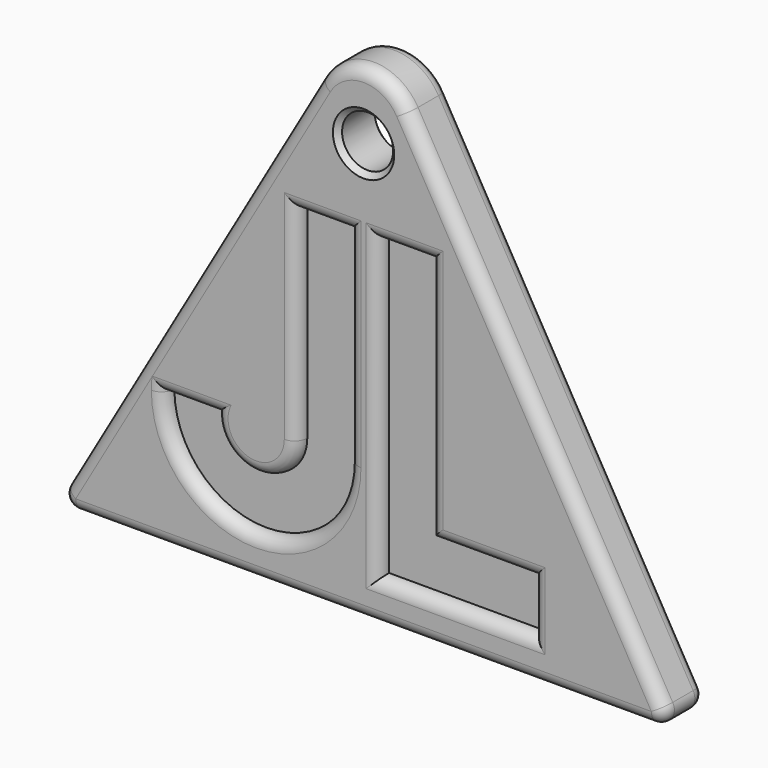
from build123d import *

# Parameters (mm, degrees)
F2_DEPTH      = 10
F3_START      = 7.5
F1_W          = 20
F1_H          = 10
F3_DEPTH      = 17.5
F4_W          = 20
F4_H          = 10
F5_DEPTH      = 2.5
F6_T1_DEPTH   = 5
F6_T3_DEPTH   = 123.1634295109
F6_T5_DEPTH   = 112.583302492
F6_T7_DEPTH   = 123.1634295109
F6_T9_DEPTH   = 54.25
F6_T11_DEPTH  = 26.25
F6_T13_DEPTH  = 10
F6_T15_DEPTH  = 30
F6_T17_DEPTH  = 58
F6_T19_DEPTH  = 10
F6_T21_DEPTH  = 40
F6_T23_DEPTH  = 10
F6_T25_DEPTH  = 30
F6_T27_DEPTH  = 26.25
F6_T32_DEPTH  = 2.5
F6_T38_DEPTH  = 2.5
F6_T44_DEPTH  = 2.5
F6_T50_DEPTH  = 2.5
F6_T56_DEPTH  = 16.25
F6_T61_DEPTH  = 22.5
F6_S62_R      = 8
F6_T63_DEPTH  = 13
F6_S64_R      = 18
F6_T65_DEPTH  = 13
F6_T67_ANGLE  = 180
F6_T71_DEPTH  = 16.25
F6_T74_ANGLE  = 180
F6_T78_DEPTH  = 16.25
F6_T81_ANGLE  = 180
F6_T85_DEPTH  = 22.5
F6_S86_R      = 8
F6_T87_DEPTH  = 13
F6_S88_R      = 18
F6_T89_DEPTH  = 13
F6_T91_ANGLE  = 180
F6_T95_DEPTH  = 16.25
F6_T101_DEPTH = 60.5
F6_T105_DEPTH = 16.25
F6_T112_DEPTH = 32.5
F6_T116_DEPTH = 16.25
F6_T123_DEPTH = 16.25
F6_T127_DEPTH = 36.25
F6_T134_DEPTH = 36.25
F6_T138_DEPTH = 64.25
F6_T145_DEPTH = 64.25
F6_T149_DEPTH = 16.25
F6_T157_DEPTH = 22.5
F6_S158_R     = 8
F6_T159_DEPTH = 13
F6_T162_ANGLE = 224.8343140314
F6_T169_DEPTH = 22.5
F6_S170_R     = 18
F6_T171_DEPTH = 13
F6_T174_ANGLE = 199.9263617918
F6_T181_DEPTH = 46.25
F6_T185_DEPTH = 16.25
F6_T192_DEPTH = 16.25
F6_T197_DEPTH = 46.25
F6_T204_DEPTH = 46.25
F6_T208_DEPTH = 16.25
F6_T216_DEPTH = 16.25
F6_T220_DEPTH = 46.25
F6_T227_ANGLE = 224.8343140314
F6_T231_DEPTH = 22.5
F6_S232_R     = 8
F6_T233_DEPTH = 13
F6_T239_DEPTH = 22.5
F6_S240_R     = 18
F6_T241_DEPTH = 13
F6_T244_ANGLE = 199.9263617918
F6_T251_DEPTH = 64.25
F6_T255_DEPTH = 36.25
F6_T262_DEPTH = 64.25
F6_T266_DEPTH = 16.25
F6_T274_DEPTH = 36.25
F6_T278_DEPTH = 16.25
F6_T285_DEPTH = 16.25
F6_T289_DEPTH = 32.5
F6_T296_DEPTH = 60.5
F6_T300_DEPTH = 16.25
F7_R          = 5
F8_DEPTH      = 25
F9_SIZE       = 1
F10_T1_DEPTH  = 9.9999999998
F10_T4_ANGLE  = 120
F10_T6_ANGLE  = 120


# Not quite as in the source:
# - a fillet or chamfer that OpenCascade refuses, or shapes differently, is made with other operations: its cross-section is extruded or revolved along the edge and cut away or added


with BuildPart() as f2:
    # F0 (on Front) → F2 (new body)
    with BuildSketch(Plane.XZ):
        Polygon((60.6217782649, -35), (0, 70), (-60.6217782649, -35), align=None)
    extrude(amount=F2_DEPTH)

    # F1 (on Front) → F3 (cut)
    with BuildSketch(Plane.XZ.offset(F3_START)):
        with BuildLine():
            ThreePointArc((-39, -9), (-21, -27), (-3, -9))
            Line((-3, -9), (-3, 31))
            Line((-3, 31), (-13, 31))
            Line((-13, 31), (-13, -9))
            ThreePointArc((-13, -9), (-21, -17), (-29, -9))
            Line((-29, -9), (-39, -9))
        make_face()
        Polygon((13, 31), (3, 31), (3, -27), (13, -27), (13, -17), align=None)
        with Locations((23, -22)):
            Rectangle(F1_W, F1_H)
    extrude(amount=F3_DEPTH, mode=Mode.SUBTRACT)

    # F4 (on face) → F5 (cut)
    with BuildSketch(Plane(origin=(0, 0, 0), x_dir=(-1, 0, 0), z_dir=(0, 1, 0))):
        with BuildLine():
            ThreePointArc((-39, -9), (-21, -27), (-3, -9))
            Line((-3, -9), (-3, 31))
            Line((-3, 31), (-13, 31))
            Line((-13, 31), (-13, -9))
            ThreePointArc((-13, -9), (-21, -17), (-29, -9))
            Line((-29, -9), (-39, -9))
        make_face()
        Polygon((13, 31), (3, 31), (3, -27), (13, -27), (13, -17), align=None)
        with Locations((23, -22)):
            Rectangle(F4_W, F4_H)
    extrude(amount=-F5_DEPTH, mode=Mode.SUBTRACT)

    # F6: fillet of radius 2.5 on 32 edges, made by hand

    # F6_s2 → F6_t1 (cut)
    with BuildSketch(Plane.XZ.offset(2.5)):
        with BuildLine():
            ThreePointArc((58.4567147554, -31.25), (58.4567147554, -33.75), (56.291651246, -35))
            Line((56.291651246, -35), (60.6217782649, -35))
            Line((60.6217782649, -35), (58.4567147554, -31.25))
        make_face()
        with BuildLine():
            ThreePointArc((-56.291651246, -35), (-58.4567147554, -33.75), (-58.4567147554, -31.25))
            Line((-58.4567147554, -31.25), (-60.6217782649, -35))
            Line((-60.6217782649, -35), (-56.291651246, -35))
        make_face()
    extrude(amount=F6_T1_DEPTH, mode=Mode.SUBTRACT)

    # F6_s4 → F6_t3 (cut)
    with BuildSketch(Plane(origin=(28.145825623, 0, -48.75), x_dir=(0, 1, 0), z_dir=(-0.5, 0, 0.8660254038))):
        with BuildLine():
            ThreePointArc((-2.5, -35), (-0.732233047, -34.267766953), (0, -32.5))
            Line((0, -32.5), (0, -35))
            Line((0, -35), (-2.5, -35))
        make_face()
        with BuildLine():
            ThreePointArc((-7.5, -35), (-9.267766953, -34.267766953), (-10, -32.5))
            Line((-10, -32.5), (-10, -35))
            Line((-10, -35), (-7.5, -35))
        make_face()
    extrude(amount=F6_T3_DEPTH, mode=Mode.SUBTRACT)

    # F6_s6 → F6_t5 (cut)
    with BuildSketch(Plane.YZ.offset(-56.291651246)):
        with BuildLine():
            ThreePointArc((-2.5, -35), (-0.732233047, -34.267766953), (0, -32.5))
            Line((0, -32.5), (0, -35))
            Line((0, -35), (-2.5, -35))
        make_face()
        with BuildLine():
            ThreePointArc((-7.5, -35), (-9.267766953, -34.267766953), (-10, -32.5))
            Line((-10, -32.5), (-10, -35))
            Line((-10, -35), (-7.5, -35))
        make_face()
    extrude(amount=F6_T5_DEPTH, mode=Mode.SUBTRACT)

    # F6_s8 → F6_t7 (cut)
    with BuildSketch(Plane(origin=(33.4358891325, 0, 57.9126587737), x_dir=(0, 1, 0), z_dir=(-0.5, 0, -0.8660254038))):
        with BuildLine():
            ThreePointArc((-2.5, -35), (-0.732233047, -34.267766953), (0, -32.5))
            Line((0, -32.5), (0, -35))
            Line((0, -35), (-2.5, -35))
        make_face()
        with BuildLine():
            ThreePointArc((-7.5, -35), (-9.267766953, -34.267766953), (-10, -32.5))
            Line((-10, -32.5), (-10, -35))
            Line((-10, -35), (-7.5, -35))
        make_face()
    extrude(amount=F6_T7_DEPTH, mode=Mode.SUBTRACT)

    # F6_s10 → F6_t9 (cut)
    with BuildSketch(Plane.XY.offset(-23.25)):
        with BuildLine():
            ThreePointArc((-15.5, 0), (-13.732233047, -0.732233047), (-13, -2.5))
            Line((-13, -2.5), (-13, 0))
            Line((-13, 0), (-15.5, 0))
        make_face()
        with BuildLine():
            ThreePointArc((15.5, -10), (13.732233047, -9.267766953), (13, -7.5))
            Line((13, -7.5), (13, -10))
            Line((13, -10), (15.5, -10))
        make_face()
    extrude(amount=F6_T9_DEPTH, mode=Mode.SUBTRACT)

    # F6_s12 → F6_t11 (cut)
    with BuildSketch(Plane.YZ.offset(-33)):
        with BuildLine():
            ThreePointArc((0, -14.5), (-0.732233047, -16.267766953), (-2.5, -17))
            Line((-2.5, -17), (0, -17))
            Line((0, -17), (0, -14.5))
        make_face()
    extrude(amount=F6_T11_DEPTH, mode=Mode.SUBTRACT)

    # F6_s14 → F6_t13 (cut)
    with BuildSketch(Plane.XY.offset(-27)):
        with BuildLine():
            ThreePointArc((-35.5, 0), (-33.732233047, -0.732233047), (-33, -2.5))
            Line((-33, -2.5), (-33, 0))
            Line((-33, 0), (-35.5, 0))
        make_face()
        with BuildLine():
            ThreePointArc((35.5, -10), (33.732233047, -9.267766953), (33, -7.5))
            Line((33, -7.5), (33, -10))
            Line((33, -10), (35.5, -10))
        make_face()
    extrude(amount=F6_T13_DEPTH, mode=Mode.SUBTRACT)

    # F6_s16 → F6_t15 (cut)
    with BuildSketch(Plane.YZ.offset(-33)):
        with BuildLine():
            ThreePointArc((0, -29.5), (-0.732233047, -27.732233047), (-2.5, -27))
            Line((-2.5, -27), (0, -27))
            Line((0, -27), (0, -29.5))
        make_face()
    extrude(amount=F6_T15_DEPTH, mode=Mode.SUBTRACT)

    # F6_s18 → F6_t17 (cut)
    with BuildSketch(Plane.XY.offset(-27)):
        with BuildLine():
            ThreePointArc((-0.5, 0), (-2.267766953, -0.732233047), (-3, -2.5))
            Line((-3, -2.5), (-3, 0))
            Line((-3, 0), (-0.5, 0))
        make_face()
        with BuildLine():
            ThreePointArc((0.5, -10), (2.267766953, -9.267766953), (3, -7.5))
            Line((3, -7.5), (3, -10))
            Line((3, -10), (0.5, -10))
        make_face()
    extrude(amount=F6_T17_DEPTH, mode=Mode.SUBTRACT)

    # F6_s20 → F6_t19 (cut)
    with BuildSketch(Plane.YZ.offset(-13)):
        with BuildLine():
            ThreePointArc((0, 33.5), (-0.732233047, 31.732233047), (-2.5, 31))
            Line((-2.5, 31), (0, 31))
            Line((0, 31), (0, 33.5))
        make_face()
        with BuildLine():
            ThreePointArc((-10, 33.5), (-9.267766953, 31.732233047), (-7.5, 31))
            Line((-7.5, 31), (-10, 31))
            Line((-10, 31), (-10, 33.5))
        make_face()
    extrude(amount=F6_T19_DEPTH, mode=Mode.SUBTRACT)

    # F6_s22 → F6_t21 (cut)
    with BuildSketch(Plane.XY.offset(-9)):
        with BuildLine():
            ThreePointArc((15.5, 0), (13.732233047, -0.732233047), (13, -2.5))
            Line((13, -2.5), (13, 0))
            Line((13, 0), (15.5, 0))
        make_face()
        with BuildLine():
            ThreePointArc((0.5, 0), (2.267766953, -0.732233047), (3, -2.5))
            Line((3, -2.5), (3, 0))
            Line((3, 0), (0.5, 0))
        make_face()
        with BuildLine():
            ThreePointArc((-0.5, -10), (-2.267766953, -9.267766953), (-3, -7.5))
            Line((-3, -7.5), (-3, -10))
            Line((-3, -10), (-0.5, -10))
        make_face()
        with BuildLine():
            ThreePointArc((-15.5, -10), (-13.732233047, -9.267766953), (-13, -7.5))
            Line((-13, -7.5), (-13, -10))
            Line((-13, -10), (-15.5, -10))
        make_face()
    extrude(amount=F6_T21_DEPTH, mode=Mode.SUBTRACT)

    # F6_s24 → F6_t23 (cut)
    with BuildSketch(Plane.YZ.offset(3)):
        with BuildLine():
            ThreePointArc((0, 33.5), (-0.732233047, 31.732233047), (-2.5, 31))
            Line((-2.5, 31), (0, 31))
            Line((0, 31), (0, 33.5))
        make_face()
        with BuildLine():
            ThreePointArc((-10, 33.5), (-9.267766953, 31.732233047), (-7.5, 31))
            Line((-7.5, 31), (-10, 31))
            Line((-10, 31), (-10, 33.5))
        make_face()
    extrude(amount=F6_T23_DEPTH, mode=Mode.SUBTRACT)

    # F6_s26 → F6_t25 (cut)
    with BuildSketch(Plane.YZ.offset(3)):
        with BuildLine():
            ThreePointArc((-10, -29.5), (-9.267766953, -27.732233047), (-7.5, -27))
            Line((-7.5, -27), (-10, -27))
            Line((-10, -27), (-10, -29.5))
        make_face()
    extrude(amount=F6_T25_DEPTH, mode=Mode.SUBTRACT)

    # F6_s28 → F6_t27 (cut)
    with BuildSketch(Plane.YZ.offset(6.75)):
        with BuildLine():
            ThreePointArc((-10, -14.5), (-9.267766953, -16.267766953), (-7.5, -17))
            Line((-7.5, -17), (-10, -17))
            Line((-10, -17), (-10, -14.5))
        make_face()
    extrude(amount=F6_T27_DEPTH, mode=Mode.SUBTRACT)


with BuildPart() as f6_tool30:
    # F6_s31 → F6_t32 (new body)
    with BuildSketch(Plane.XZ.offset(2.5)):
        Polygon((56.291651246, -32.5), (58.4567147554, -31.25), (60.6217782649, -35), (56.291651246, -35), align=None)
    extrude(amount=-F6_T32_DEPTH)

    # F6_s33 → F6_t34 (revolve, cut)
    with BuildSketch(Plane(origin=(56.291651246, -2.5, -32.5), x_dir=(-0.8660254038, 0, 0.5), z_dir=(-0.5, 0, -0.8660254038))):
        with BuildLine():
            ThreePointArc((0, -2.5), (2.5, 0), (0, 2.5))
            Line((0, 2.5), (0, -2.5))
        make_face()
    revolve(axis=Axis((56.291651246, -2.5, -32.5), (0, 1, 0)), mode=Mode.SUBTRACT)


with BuildPart() as f2_1:
    add(f2.part)

    # F6_t29: cut F6_tool30
    add(f6_tool30.part, mode=Mode.SUBTRACT)


with BuildPart() as f6_tool36:
    # F6_s37 → F6_t38 (new body)
    with BuildSketch(Plane.XZ.offset(7.5)):
        Polygon((56.291651246, -32.5), (58.4567147554, -31.25), (60.6217782649, -35), (56.291651246, -35), align=None)
    extrude(amount=F6_T38_DEPTH)

    # F6_s39 → F6_t40 (revolve, cut)
    with BuildSketch(Plane(origin=(56.291651246, -7.5, -32.5), x_dir=(-0.8660254038, 0, 0.5), z_dir=(0.5, 0, 0.8660254038))):
        with BuildLine():
            ThreePointArc((0, -2.5), (2.5, 0), (0, 2.5))
            Line((0, 2.5), (0, -2.5))
        make_face()
    revolve(axis=Axis((56.291651246, -7.5, -32.5), (0, -1, 0)), mode=Mode.SUBTRACT)


with BuildPart() as f2_2:
    add(f2_1.part)

    # F6_t35: cut F6_tool36
    add(f6_tool36.part, mode=Mode.SUBTRACT)


with BuildPart() as f6_tool42:
    # F6_s43 → F6_t44 (new body)
    with BuildSketch(Plane.XZ.offset(2.5)):
        Polygon((-56.291651246, -32.5), (-56.291651246, -35), (-60.6217782649, -35), (-58.4567147554, -31.25), align=None)
    extrude(amount=-F6_T44_DEPTH)

    # F6_s45 → F6_t46 (revolve, cut)
    with BuildSketch(Plane(origin=(-56.291651246, -2.5, -32.5), x_dir=(0.8660254038, 0, 0.5), z_dir=(-0.5, 0, 0.8660254038))):
        with BuildLine():
            ThreePointArc((0, -2.5), (2.5, 0), (0, 2.5))
            Line((0, 2.5), (0, -2.5))
        make_face()
    revolve(axis=Axis((-56.291651246, -2.5, -32.5), (0, 1, 0)), mode=Mode.SUBTRACT)


with BuildPart() as f2_3:
    add(f2_2.part)

    # F6_t41: cut F6_tool42
    add(f6_tool42.part, mode=Mode.SUBTRACT)


with BuildPart() as f6_tool48:
    # F6_s49 → F6_t50 (new body)
    with BuildSketch(Plane.XZ.offset(7.5)):
        Polygon((-56.291651246, -32.5), (-56.291651246, -35), (-60.6217782649, -35), (-58.4567147554, -31.25), align=None)
    extrude(amount=F6_T50_DEPTH)

    # F6_s51 → F6_t52 (revolve, cut)
    with BuildSketch(Plane(origin=(-56.291651246, -7.5, -32.5), x_dir=(0.8660254038, 0, 0.5), z_dir=(0.5, 0, -0.8660254038))):
        with BuildLine():
            ThreePointArc((0, -2.5), (2.5, 0), (0, 2.5))
            Line((0, 2.5), (0, -2.5))
        make_face()
    revolve(axis=Axis((-56.291651246, -7.5, -32.5), (0, -1, 0)), mode=Mode.SUBTRACT)


with BuildPart() as f2_4:
    add(f2_3.part)

    # F6_t47: cut F6_tool48
    add(f6_tool48.part, mode=Mode.SUBTRACT)


with BuildPart() as f6_tool54:
    # F6_s55 → F6_t56 (new body)
    with BuildSketch(Plane.YZ.offset(-13)):
        with BuildLine():
            ThreePointArc((0, 33.5), (-0.732233047, 31.732233047), (-2.5, 31))
            Line((-2.5, 31), (0, 31))
            Line((0, 31), (0, 33.5))
        make_face()
    extrude(amount=F6_T56_DEPTH)

    split(bisect_by=Plane.YZ.offset(3), keep=Keep.TOP)


with BuildPart() as f2_5:
    add(f2_4.part)

    # F6_t53: cut F6_tool54
    add(f6_tool54.part, mode=Mode.SUBTRACT)


with BuildPart() as f6_tool59:
    # F6_s60 → F6_t61 (new body)
    with BuildSketch(Plane.YZ.offset(22.75)):
        with BuildLine():
            ThreePointArc((0, -6.5), (-0.732233047, -8.267766953), (-2.5, -9))
            Line((-2.5, -9), (0, -9))
            Line((0, -9), (0, -6.5))
        make_face()
    extrude(amount=F6_T61_DEPTH)

    # F6_s62 → F6_t63 (cut, symmetric)
    with BuildSketch(Plane.XZ.offset(1.2)):
        with Locations((21, -9)):
            Circle(F6_S62_R)
    extrude(amount=F6_T63_DEPTH, both=True, mode=Mode.SUBTRACT)

    # F6_s64 → F6_t65 (intersect, symmetric)
    with BuildSketch(Plane.XZ.offset(1.2)):
        with Locations((21, -9)):
            Circle(F6_S64_R)
    extrude(amount=F6_T65_DEPTH, both=True, mode=Mode.INTERSECT)


with BuildPart() as f2_6:
    add(f2_5.part)

    # F6_t58: cut F6_tool59
    add(f6_tool59.part, mode=Mode.SUBTRACT)

    # F6_s66 → F6_t67 (revolve, cut)
    with BuildSketch(Plane.XY.offset(-9)):
        with BuildLine():
            ThreePointArc((15.5, 0), (13.732233047, -0.732233047), (13, -2.5))
            Line((13, -2.5), (13, 0))
            Line((13, 0), (15.5, 0))
        make_face()
    revolve(axis=Axis((21, 0, -9), (0, -1, 0)), revolution_arc=F6_T67_ANGLE, mode=Mode.SUBTRACT)


with BuildPart() as f6_tool69:
    # F6_s70 → F6_t71 (new body)
    with BuildSketch(Plane.YZ.offset(-3.25)):
        with BuildLine():
            ThreePointArc((0, 33.5), (-0.732233047, 31.732233047), (-2.5, 31))
            Line((-2.5, 31), (0, 31))
            Line((0, 31), (0, 33.5))
        make_face()
    extrude(amount=F6_T71_DEPTH)

    split(bisect_by=Plane.YZ.offset(-3), keep=Keep.BOTTOM)


with BuildPart() as f2_7:
    add(f2_6.part)

    # F6_t68: cut F6_tool69
    add(f6_tool69.part, mode=Mode.SUBTRACT)

    # F6_s73 → F6_t74 (revolve, cut)
    with BuildSketch(Plane.XY.offset(-9)):
        with BuildLine():
            ThreePointArc((41.5, 0), (39.732233047, -0.732233047), (39, -2.5))
            Line((39, -2.5), (39, 0))
            Line((39, 0), (41.5, 0))
        make_face()
    revolve(axis=Axis((21, 0, -9), (0, 1, 0)), revolution_arc=F6_T74_ANGLE, mode=Mode.SUBTRACT)


with BuildPart() as f6_tool76:
    # F6_s77 → F6_t78 (new body)
    with BuildSketch(Plane.YZ.offset(-13)):
        with BuildLine():
            ThreePointArc((-10, 33.5), (-9.267766953, 31.732233047), (-7.5, 31))
            Line((-7.5, 31), (-10, 31))
            Line((-10, 31), (-10, 33.5))
        make_face()
    extrude(amount=F6_T78_DEPTH)

    split(bisect_by=Plane.YZ.offset(3), keep=Keep.TOP)


with BuildPart() as f2_8:
    add(f2_7.part)

    # F6_t75: cut F6_tool76
    add(f6_tool76.part, mode=Mode.SUBTRACT)

    # F6_s80 → F6_t81 (revolve, cut)
    with BuildSketch(Plane.XY.offset(-9)):
        with BuildLine():
            ThreePointArc((-15.5, -10), (-13.732233047, -9.267766953), (-13, -7.5))
            Line((-13, -7.5), (-13, -10))
            Line((-13, -10), (-15.5, -10))
        make_face()
    revolve(axis=Axis((-21, -10, -9), (0, 1, 0)), revolution_arc=F6_T81_ANGLE, mode=Mode.SUBTRACT)


with BuildPart() as f6_tool83:
    # F6_s84 → F6_t85 (new body)
    with BuildSketch(Plane.YZ.offset(-45.25)):
        with BuildLine():
            ThreePointArc((-10, -6.5), (-9.267766953, -8.267766953), (-7.5, -9))
            Line((-7.5, -9), (-10, -9))
            Line((-10, -9), (-10, -6.5))
        make_face()
    extrude(amount=F6_T85_DEPTH)

    # F6_s86 → F6_t87 (cut, symmetric)
    with BuildSketch(Plane.XZ.offset(8.8)):
        with Locations((-21, -9)):
            Circle(F6_S86_R)
    extrude(amount=F6_T87_DEPTH, both=True, mode=Mode.SUBTRACT)

    # F6_s88 → F6_t89 (intersect, symmetric)
    with BuildSketch(Plane.XZ.offset(8.8)):
        with Locations((-21, -9)):
            Circle(F6_S88_R)
    extrude(amount=F6_T89_DEPTH, both=True, mode=Mode.INTERSECT)


with BuildPart() as f2_9:
    add(f2_8.part)

    # F6_t82: cut F6_tool83
    add(f6_tool83.part, mode=Mode.SUBTRACT)

    # F6_s90 → F6_t91 (revolve, cut)
    with BuildSketch(Plane.XY.offset(-9)):
        with BuildLine():
            ThreePointArc((-0.5, -10), (-2.267766953, -9.267766953), (-3, -7.5))
            Line((-3, -7.5), (-3, -10))
            Line((-3, -10), (-0.5, -10))
        make_face()
    revolve(axis=Axis((-21, -10, -9), (0, 1, 0)), revolution_arc=F6_T91_ANGLE, mode=Mode.SUBTRACT)


with BuildPart() as f6_tool93:
    # F6_s94 → F6_t95 (new body)
    with BuildSketch(Plane.YZ.offset(-3.25)):
        with BuildLine():
            ThreePointArc((-10, 33.5), (-9.267766953, 31.732233047), (-7.5, 31))
            Line((-7.5, 31), (-10, 31))
            Line((-10, 31), (-10, 33.5))
        make_face()
    extrude(amount=F6_T95_DEPTH)

    split(bisect_by=Plane.YZ.offset(-3), keep=Keep.BOTTOM)


with BuildPart() as f2_10:
    add(f2_9.part)

    # F6_t92: cut F6_tool93
    add(f6_tool93.part, mode=Mode.SUBTRACT)


with BuildPart() as f6_tool99:
    # F6_s100 → F6_t101 (new body)
    with BuildSketch(Plane.XY.offset(-23.25)):
        with BuildLine():
            ThreePointArc((-15.5, 0), (-13.732233047, -0.732233047), (-13, -2.5))
            Line((-13, -2.5), (-13, 0))
            Line((-13, 0), (-15.5, 0))
        make_face()
    extrude(amount=F6_T101_DEPTH)

    split(bisect_by=Plane.XY.offset(31), keep=Keep.TOP)


with BuildPart() as f6_tool103:
    # F6_s104 → F6_t105 (new body)
    with BuildSketch(Plane.YZ.offset(-19.25)):
        with BuildLine():
            ThreePointArc((0, 33.5), (-0.732233047, 31.732233047), (-2.5, 31))
            Line((-2.5, 31), (0, 31))
            Line((0, 31), (0, 33.5))
        make_face()
    extrude(amount=F6_T105_DEPTH)

    split(bisect_by=Plane.YZ.offset(-13), keep=Keep.BOTTOM)


with BuildPart() as f6_tool99_1:
    add(f6_tool99.part)

    # F6_t107: intersect F6_tool103
    add(f6_tool103.part, mode=Mode.INTERSECT)


with BuildPart() as f2_11:
    add(f2_10.part)

    # F6_t97: cut F6_tool99
    add(f6_tool99_1.part, mode=Mode.SUBTRACT)


with BuildPart() as f6_tool110:
    # F6_s111 → F6_t112 (new body)
    with BuildSketch(Plane.YZ.offset(-39.25)):
        with BuildLine():
            ThreePointArc((0, -14.5), (-0.732233047, -16.267766953), (-2.5, -17))
            Line((-2.5, -17), (0, -17))
            Line((0, -17), (0, -14.5))
        make_face()
    extrude(amount=F6_T112_DEPTH)

    split(bisect_by=Plane.YZ.offset(-33), keep=Keep.BOTTOM)


with BuildPart() as f6_tool114:
    # F6_s115 → F6_t116 (new body)
    with BuildSketch(Plane.XY.offset(-27)):
        with BuildLine():
            ThreePointArc((-35.5, 0), (-33.732233047, -0.732233047), (-33, -2.5))
            Line((-33, -2.5), (-33, 0))
            Line((-33, 0), (-35.5, 0))
        make_face()
    extrude(amount=F6_T116_DEPTH)

    split(bisect_by=Plane.XY.offset(-17), keep=Keep.TOP)


with BuildPart() as f6_tool110_1:
    add(f6_tool110.part)

    # F6_t118: intersect F6_tool114
    add(f6_tool114.part, mode=Mode.INTERSECT)


with BuildPart() as f2_12:
    add(f2_11.part)

    # F6_t108: cut F6_tool110
    add(f6_tool110_1.part, mode=Mode.SUBTRACT)


with BuildPart() as f6_tool121:
    # F6_s122 → F6_t123 (new body)
    with BuildSketch(Plane.XY.offset(-33.25)):
        with BuildLine():
            ThreePointArc((-35.5, 0), (-33.732233047, -0.732233047), (-33, -2.5))
            Line((-33, -2.5), (-33, 0))
            Line((-33, 0), (-35.5, 0))
        make_face()
    extrude(amount=F6_T123_DEPTH)

    split(bisect_by=Plane.XY.offset(-27), keep=Keep.BOTTOM)


with BuildPart() as f6_tool125:
    # F6_s126 → F6_t127 (new body)
    with BuildSketch(Plane.YZ.offset(-3)):
        with BuildLine():
            ThreePointArc((0, -29.5), (-0.732233047, -27.732233047), (-2.5, -27))
            Line((-2.5, -27), (0, -27))
            Line((0, -27), (0, -29.5))
        make_face()
    extrude(amount=-F6_T127_DEPTH)

    split(bisect_by=Plane.YZ.offset(-33), keep=Keep.BOTTOM)


with BuildPart() as f6_tool121_1:
    add(f6_tool121.part)

    # F6_t129: intersect F6_tool125
    add(f6_tool125.part, mode=Mode.INTERSECT)


with BuildPart() as f2_13:
    add(f2_12.part)

    # F6_t119: cut F6_tool121
    add(f6_tool121_1.part, mode=Mode.SUBTRACT)


with BuildPart() as f6_tool132:
    # F6_s133 → F6_t134 (new body)
    with BuildSketch(Plane.YZ.offset(3.25)):
        with BuildLine():
            ThreePointArc((0, -29.5), (-0.732233047, -27.732233047), (-2.5, -27))
            Line((-2.5, -27), (0, -27))
            Line((0, -27), (0, -29.5))
        make_face()
    extrude(amount=-F6_T134_DEPTH)

    split(bisect_by=Plane.YZ.offset(-3), keep=Keep.TOP)


with BuildPart() as f6_tool136:
    # F6_s137 → F6_t138 (new body)
    with BuildSketch(Plane.XY.offset(31)):
        with BuildLine():
            ThreePointArc((-0.5, 0), (-2.267766953, -0.732233047), (-3, -2.5))
            Line((-3, -2.5), (-3, 0))
            Line((-3, 0), (-0.5, 0))
        make_face()
    extrude(amount=-F6_T138_DEPTH)

    split(bisect_by=Plane.XY.offset(-27), keep=Keep.BOTTOM)


with BuildPart() as f6_tool132_1:
    add(f6_tool132.part)

    # F6_t140: intersect F6_tool136
    add(f6_tool136.part, mode=Mode.INTERSECT)


with BuildPart() as f2_14:
    add(f2_13.part)

    # F6_t130: cut F6_tool132
    add(f6_tool132_1.part, mode=Mode.SUBTRACT)


with BuildPart() as f6_tool143:
    # F6_s144 → F6_t145 (new body)
    with BuildSketch(Plane.XY.offset(37.25)):
        with BuildLine():
            ThreePointArc((-0.5, 0), (-2.267766953, -0.732233047), (-3, -2.5))
            Line((-3, -2.5), (-3, 0))
            Line((-3, 0), (-0.5, 0))
        make_face()
    extrude(amount=-F6_T145_DEPTH)

    split(bisect_by=Plane.XY.offset(31), keep=Keep.TOP)


with BuildPart() as f6_tool147:
    # F6_s148 → F6_t149 (new body)
    with BuildSketch(Plane.YZ.offset(-13)):
        with BuildLine():
            ThreePointArc((0, 33.5), (-0.732233047, 31.732233047), (-2.5, 31))
            Line((-2.5, 31), (0, 31))
            Line((0, 31), (0, 33.5))
        make_face()
    extrude(amount=F6_T149_DEPTH)

    split(bisect_by=Plane.YZ.offset(-3), keep=Keep.TOP)

    split(bisect_by=Plane.YZ.offset(3), keep=Keep.BOTTOM)


with BuildPart() as f6_tool143_1:
    add(f6_tool143.part)

    # F6_t152: intersect F6_tool147
    add(f6_tool147.part, mode=Mode.INTERSECT)


with BuildPart() as f2_15:
    add(f2_14.part)

    # F6_t141: cut F6_tool143
    add(f6_tool143_1.part, mode=Mode.SUBTRACT)


with BuildPart() as f6_tool155:
    # F6_s156 → F6_t157 (new body)
    with BuildSketch(Plane.YZ.offset(22.75)):
        with BuildLine():
            ThreePointArc((0, -6.5), (-0.732233047, -8.267766953), (-2.5, -9))
            Line((-2.5, -9), (0, -9))
            Line((0, -9), (0, -6.5))
        make_face()
    extrude(amount=F6_T157_DEPTH)

    # F6_s158 → F6_t159 (intersect, symmetric)
    with BuildSketch(Plane.XZ.offset(1.2)):
        with Locations((21, -9)):
            Circle(F6_S158_R)
    extrude(amount=F6_T159_DEPTH, both=True, mode=Mode.INTERSECT)


with BuildPart() as f6_tool160:
    # F6_s161 → F6_t162 (revolve)
    with BuildSketch(Plane.XY.offset(-9)):
        with BuildLine():
            ThreePointArc((15.5, 0), (13.732233047, -0.732233047), (13, -2.5))
            Line((13, -2.5), (13, 0))
            Line((13, 0), (15.5, 0))
        make_face()
    revolve(axis=Axis((21, 0, -9), (0, -1, 0)), revolution_arc=F6_T162_ANGLE)

    split(bisect_by=Plane.XY.offset(-9), keep=Keep.TOP)


with BuildPart() as f6_tool155_1:
    add(f6_tool155.part)

    # F6_t164: intersect F6_tool160
    add(f6_tool160.part, mode=Mode.INTERSECT)


with BuildPart() as f2_16:
    add(f2_15.part)

    # F6_t153: cut F6_tool155
    add(f6_tool155_1.part, mode=Mode.SUBTRACT)


with BuildPart() as f6_tool167:
    # F6_s168 → F6_t169 (new body)
    with BuildSketch(Plane.YZ.offset(22.75)):
        with BuildLine():
            ThreePointArc((0, -6.5), (-0.732233047, -8.267766953), (-2.5, -9))
            Line((-2.5, -9), (0, -9))
            Line((0, -9), (0, -6.5))
        make_face()
    extrude(amount=F6_T169_DEPTH)

    # F6_s170 → F6_t171 (cut, symmetric)
    with BuildSketch(Plane.XZ.offset(1.2)):
        with Locations((21, -9)):
            Circle(F6_S170_R)
    extrude(amount=F6_T171_DEPTH, both=True, mode=Mode.SUBTRACT)


with BuildPart() as f6_tool172:
    # F6_s173 → F6_t174 (revolve)
    with BuildSketch(Plane(origin=(5.322885035, 0, -14.6831959933), x_dir=(0, 1, 0), z_dir=(-0.3408121408, 0, 0.9401314188))):
        with BuildLine():
            ThreePointArc((0, -37.1754505284), (-0.732233047, -35.4076835755), (-2.5, -34.6754505284))
            Line((-2.5, -34.6754505284), (0, -34.6754505284))
            Line((0, -34.6754505284), (0, -37.1754505284))
        make_face()
    revolve(axis=Axis((21, 0, -9), (0, 1, 0)), revolution_arc=F6_T174_ANGLE)

    split(bisect_by=Plane.XY.offset(-9), keep=Keep.TOP)


with BuildPart() as f6_tool167_1:
    add(f6_tool167.part)

    # F6_t176: intersect F6_tool172
    add(f6_tool172.part, mode=Mode.INTERSECT)


with BuildPart() as f2_17:
    add(f2_16.part)

    # F6_t165: cut F6_tool167
    add(f6_tool167_1.part, mode=Mode.SUBTRACT)


with BuildPart() as f6_tool179:
    # F6_s180 → F6_t181 (new body)
    with BuildSketch(Plane.XY.offset(37.25)):
        with BuildLine():
            ThreePointArc((15.5, 0), (13.732233047, -0.732233047), (13, -2.5))
            Line((13, -2.5), (13, 0))
            Line((13, 0), (15.5, 0))
        make_face()
    extrude(amount=-F6_T181_DEPTH)

    split(bisect_by=Plane.XY.offset(31), keep=Keep.TOP)


with BuildPart() as f6_tool183:
    # F6_s184 → F6_t185 (new body)
    with BuildSketch(Plane.YZ.offset(3)):
        with BuildLine():
            ThreePointArc((0, 33.5), (-0.732233047, 31.732233047), (-2.5, 31))
            Line((-2.5, 31), (0, 31))
            Line((0, 31), (0, 33.5))
        make_face()
    extrude(amount=F6_T185_DEPTH)

    split(bisect_by=Plane.YZ.offset(13), keep=Keep.TOP)


with BuildPart() as f6_tool179_1:
    add(f6_tool179.part)

    # F6_t187: intersect F6_tool183
    add(f6_tool183.part, mode=Mode.INTERSECT)


with BuildPart() as f2_18:
    add(f2_17.part)

    # F6_t177: cut F6_tool179
    add(f6_tool179_1.part, mode=Mode.SUBTRACT)


with BuildPart() as f6_tool190:
    # F6_s191 → F6_t192 (new body)
    with BuildSketch(Plane.YZ.offset(-3.25)):
        with BuildLine():
            ThreePointArc((0, 33.5), (-0.732233047, 31.732233047), (-2.5, 31))
            Line((-2.5, 31), (0, 31))
            Line((0, 31), (0, 33.5))
        make_face()
    extrude(amount=F6_T192_DEPTH)

    split(bisect_by=Plane.YZ.offset(-3), keep=Keep.TOP)

    split(bisect_by=Plane.YZ.offset(3), keep=Keep.BOTTOM)


with BuildPart() as f6_tool195:
    # F6_s196 → F6_t197 (new body)
    with BuildSketch(Plane.XY.offset(-9)):
        with BuildLine():
            ThreePointArc((0.5, 0), (2.267766953, -0.732233047), (3, -2.5))
            Line((3, -2.5), (3, 0))
            Line((3, 0), (0.5, 0))
        make_face()
    extrude(amount=F6_T197_DEPTH)

    split(bisect_by=Plane.XY.offset(31), keep=Keep.TOP)


with BuildPart() as f6_tool190_1:
    add(f6_tool190.part)

    # F6_t199: intersect F6_tool195
    add(f6_tool195.part, mode=Mode.INTERSECT)


with BuildPart() as f2_19:
    add(f2_18.part)

    # F6_t188: cut F6_tool190
    add(f6_tool190_1.part, mode=Mode.SUBTRACT)


with BuildPart() as f6_tool202:
    # F6_s203 → F6_t204 (new body)
    with BuildSketch(Plane.XY.offset(37.25)):
        with BuildLine():
            ThreePointArc((-0.5, -10), (-2.267766953, -9.267766953), (-3, -7.5))
            Line((-3, -7.5), (-3, -10))
            Line((-3, -10), (-0.5, -10))
        make_face()
    extrude(amount=-F6_T204_DEPTH)

    split(bisect_by=Plane.XY.offset(31), keep=Keep.TOP)


with BuildPart() as f6_tool206:
    # F6_s207 → F6_t208 (new body)
    with BuildSketch(Plane.YZ.offset(-13)):
        with BuildLine():
            ThreePointArc((-10, 33.5), (-9.267766953, 31.732233047), (-7.5, 31))
            Line((-7.5, 31), (-10, 31))
            Line((-10, 31), (-10, 33.5))
        make_face()
    extrude(amount=F6_T208_DEPTH)

    split(bisect_by=Plane.YZ.offset(-3), keep=Keep.TOP)

    split(bisect_by=Plane.YZ.offset(3), keep=Keep.BOTTOM)


with BuildPart() as f6_tool202_1:
    add(f6_tool202.part)

    # F6_t211: intersect F6_tool206
    add(f6_tool206.part, mode=Mode.INTERSECT)


with BuildPart() as f2_20:
    add(f2_19.part)

    # F6_t200: cut F6_tool202
    add(f6_tool202_1.part, mode=Mode.SUBTRACT)


with BuildPart() as f6_tool214:
    # F6_s215 → F6_t216 (new body)
    with BuildSketch(Plane.YZ.offset(-19.25)):
        with BuildLine():
            ThreePointArc((-10, 33.5), (-9.267766953, 31.732233047), (-7.5, 31))
            Line((-7.5, 31), (-10, 31))
            Line((-10, 31), (-10, 33.5))
        make_face()
    extrude(amount=F6_T216_DEPTH)

    split(bisect_by=Plane.YZ.offset(-13), keep=Keep.BOTTOM)


with BuildPart() as f6_tool218:
    # F6_s219 → F6_t220 (new body)
    with BuildSketch(Plane.XY.offset(-9)):
        with BuildLine():
            ThreePointArc((-15.5, -10), (-13.732233047, -9.267766953), (-13, -7.5))
            Line((-13, -7.5), (-13, -10))
            Line((-13, -10), (-15.5, -10))
        make_face()
    extrude(amount=F6_T220_DEPTH)

    split(bisect_by=Plane.XY.offset(31), keep=Keep.TOP)


with BuildPart() as f6_tool214_1:
    add(f6_tool214.part)

    # F6_t222: intersect F6_tool218
    add(f6_tool218.part, mode=Mode.INTERSECT)


with BuildPart() as f2_21:
    add(f2_20.part)

    # F6_t212: cut F6_tool214
    add(f6_tool214_1.part, mode=Mode.SUBTRACT)


with BuildPart() as f6_tool225:
    # F6_s226 → F6_t227 (revolve)
    with BuildSketch(Plane.XY.offset(-9)):
        with BuildLine():
            ThreePointArc((-15.5, -10), (-13.732233047, -9.267766953), (-13, -7.5))
            Line((-13, -7.5), (-13, -10))
            Line((-13, -10), (-15.5, -10))
        make_face()
    revolve(axis=Axis((-21, -10, -9), (0, 1, 0)), revolution_arc=F6_T227_ANGLE)

    split(bisect_by=Plane.XY.offset(-9), keep=Keep.TOP)


with BuildPart() as f6_tool229:
    # F6_s230 → F6_t231 (new body)
    with BuildSketch(Plane.YZ.offset(-45.25)):
        with BuildLine():
            ThreePointArc((-10, -6.5), (-9.267766953, -8.267766953), (-7.5, -9))
            Line((-7.5, -9), (-10, -9))
            Line((-10, -9), (-10, -6.5))
        make_face()
    extrude(amount=F6_T231_DEPTH)

    # F6_s232 → F6_t233 (intersect, symmetric)
    with BuildSketch(Plane.XZ.offset(8.8)):
        with Locations((-21, -9)):
            Circle(F6_S232_R)
    extrude(amount=F6_T233_DEPTH, both=True, mode=Mode.INTERSECT)


with BuildPart() as f6_tool225_1:
    add(f6_tool225.part)

    # F6_t234: intersect F6_tool229
    add(f6_tool229.part, mode=Mode.INTERSECT)


with BuildPart() as f2_22:
    add(f2_21.part)

    # F6_t223: cut F6_tool225
    add(f6_tool225_1.part, mode=Mode.SUBTRACT)


with BuildPart() as f6_tool237:
    # F6_s238 → F6_t239 (new body)
    with BuildSketch(Plane.YZ.offset(-45.25)):
        with BuildLine():
            ThreePointArc((-10, -6.5), (-9.267766953, -8.267766953), (-7.5, -9))
            Line((-7.5, -9), (-10, -9))
            Line((-10, -9), (-10, -6.5))
        make_face()
    extrude(amount=F6_T239_DEPTH)

    # F6_s240 → F6_t241 (cut, symmetric)
    with BuildSketch(Plane.XZ.offset(8.8)):
        with Locations((-21, -9)):
            Circle(F6_S240_R)
    extrude(amount=F6_T241_DEPTH, both=True, mode=Mode.SUBTRACT)


with BuildPart() as f6_tool242:
    # F6_s243 → F6_t244 (revolve)
    with BuildSketch(Plane.XY.offset(-9)):
        with BuildLine():
            ThreePointArc((-0.5, -10), (-2.267766953, -9.267766953), (-3, -7.5))
            Line((-3, -7.5), (-3, -10))
            Line((-3, -10), (-0.5, -10))
        make_face()
    revolve(axis=Axis((-21, -10, -9), (0, 1, 0)), revolution_arc=F6_T244_ANGLE)

    split(bisect_by=Plane.XY.offset(-9), keep=Keep.TOP)


with BuildPart() as f6_tool237_1:
    add(f6_tool237.part)

    # F6_t246: intersect F6_tool242
    add(f6_tool242.part, mode=Mode.INTERSECT)


with BuildPart() as f2_23:
    add(f2_22.part)

    # F6_t235: cut F6_tool237
    add(f6_tool237_1.part, mode=Mode.SUBTRACT)


with BuildPart() as f6_tool249:
    # F6_s250 → F6_t251 (new body)
    with BuildSketch(Plane.XY.offset(-33.25)):
        with BuildLine():
            ThreePointArc((0.5, -10), (2.267766953, -9.267766953), (3, -7.5))
            Line((3, -7.5), (3, -10))
            Line((3, -10), (0.5, -10))
        make_face()
    extrude(amount=F6_T251_DEPTH)

    split(bisect_by=Plane.XY.offset(-27), keep=Keep.BOTTOM)


with BuildPart() as f6_tool253:
    # F6_s254 → F6_t255 (new body)
    with BuildSketch(Plane.YZ.offset(33)):
        with BuildLine():
            ThreePointArc((-10, -29.5), (-9.267766953, -27.732233047), (-7.5, -27))
            Line((-7.5, -27), (-10, -27))
            Line((-10, -27), (-10, -29.5))
        make_face()
    extrude(amount=-F6_T255_DEPTH)

    split(bisect_by=Plane.YZ.offset(3), keep=Keep.BOTTOM)


with BuildPart() as f6_tool249_1:
    add(f6_tool249.part)

    # F6_t257: intersect F6_tool253
    add(f6_tool253.part, mode=Mode.INTERSECT)


with BuildPart() as f2_24:
    add(f2_23.part)

    # F6_t247: cut F6_tool249
    add(f6_tool249_1.part, mode=Mode.SUBTRACT)


with BuildPart() as f6_tool260:
    # F6_s261 → F6_t262 (new body)
    with BuildSketch(Plane.XY.offset(-27)):
        with BuildLine():
            ThreePointArc((0.5, -10), (2.267766953, -9.267766953), (3, -7.5))
            Line((3, -7.5), (3, -10))
            Line((3, -10), (0.5, -10))
        make_face()
    extrude(amount=F6_T262_DEPTH)

    split(bisect_by=Plane.XY.offset(31), keep=Keep.TOP)


with BuildPart() as f6_tool264:
    # F6_s265 → F6_t266 (new body)
    with BuildSketch(Plane.YZ.offset(-3.25)):
        with BuildLine():
            ThreePointArc((-10, 33.5), (-9.267766953, 31.732233047), (-7.5, 31))
            Line((-7.5, 31), (-10, 31))
            Line((-10, 31), (-10, 33.5))
        make_face()
    extrude(amount=F6_T266_DEPTH)

    split(bisect_by=Plane.YZ.offset(-3), keep=Keep.TOP)

    split(bisect_by=Plane.YZ.offset(3), keep=Keep.BOTTOM)


with BuildPart() as f6_tool260_1:
    add(f6_tool260.part)

    # F6_t269: intersect F6_tool264
    add(f6_tool264.part, mode=Mode.INTERSECT)


with BuildPart() as f2_25:
    add(f2_24.part)

    # F6_t258: cut F6_tool260
    add(f6_tool260_1.part, mode=Mode.SUBTRACT)


with BuildPart() as f6_tool272:
    # F6_s273 → F6_t274 (new body)
    with BuildSketch(Plane.YZ.offset(39.25)):
        with BuildLine():
            ThreePointArc((-10, -29.5), (-9.267766953, -27.732233047), (-7.5, -27))
            Line((-7.5, -27), (-10, -27))
            Line((-10, -27), (-10, -29.5))
        make_face()
    extrude(amount=-F6_T274_DEPTH)

    split(bisect_by=Plane.YZ.offset(33), keep=Keep.TOP)


with BuildPart() as f6_tool276:
    # F6_s277 → F6_t278 (new body)
    with BuildSketch(Plane.XY.offset(-17)):
        with BuildLine():
            ThreePointArc((35.5, -10), (33.732233047, -9.267766953), (33, -7.5))
            Line((33, -7.5), (33, -10))
            Line((33, -10), (35.5, -10))
        make_face()
    extrude(amount=-F6_T278_DEPTH)

    split(bisect_by=Plane.XY.offset(-27), keep=Keep.BOTTOM)


with BuildPart() as f6_tool272_1:
    add(f6_tool272.part)

    # F6_t280: intersect F6_tool276
    add(f6_tool276.part, mode=Mode.INTERSECT)


with BuildPart() as f2_26:
    add(f2_25.part)

    # F6_t270: cut F6_tool272
    add(f6_tool272_1.part, mode=Mode.SUBTRACT)


with BuildPart() as f6_tool283:
    # F6_s284 → F6_t285 (new body)
    with BuildSketch(Plane.XY.offset(-10.75)):
        with BuildLine():
            ThreePointArc((35.5, -10), (33.732233047, -9.267766953), (33, -7.5))
            Line((33, -7.5), (33, -10))
            Line((33, -10), (35.5, -10))
        make_face()
    extrude(amount=-F6_T285_DEPTH)

    split(bisect_by=Plane.XY.offset(-17), keep=Keep.TOP)


with BuildPart() as f6_tool287:
    # F6_s288 → F6_t289 (new body)
    with BuildSketch(Plane.YZ.offset(6.75)):
        with BuildLine():
            ThreePointArc((-10, -14.5), (-9.267766953, -16.267766953), (-7.5, -17))
            Line((-7.5, -17), (-10, -17))
            Line((-10, -17), (-10, -14.5))
        make_face()
    extrude(amount=F6_T289_DEPTH)

    split(bisect_by=Plane.YZ.offset(33), keep=Keep.TOP)


with BuildPart() as f6_tool283_1:
    add(f6_tool283.part)

    # F6_t291: intersect F6_tool287
    add(f6_tool287.part, mode=Mode.INTERSECT)


with BuildPart() as f2_27:
    add(f2_26.part)

    # F6_t281: cut F6_tool283
    add(f6_tool283_1.part, mode=Mode.SUBTRACT)


with BuildPart() as f6_tool294:
    # F6_s295 → F6_t296 (new body)
    with BuildSketch(Plane.XY.offset(37.25)):
        with BuildLine():
            ThreePointArc((15.5, -10), (13.732233047, -9.267766953), (13, -7.5))
            Line((13, -7.5), (13, -10))
            Line((13, -10), (15.5, -10))
        make_face()
    extrude(amount=-F6_T296_DEPTH)

    split(bisect_by=Plane.XY.offset(31), keep=Keep.TOP)


with BuildPart() as f6_tool298:
    # F6_s299 → F6_t300 (new body)
    with BuildSketch(Plane.YZ.offset(3)):
        with BuildLine():
            ThreePointArc((-10, 33.5), (-9.267766953, 31.732233047), (-7.5, 31))
            Line((-7.5, 31), (-10, 31))
            Line((-10, 31), (-10, 33.5))
        make_face()
    extrude(amount=F6_T300_DEPTH)

    split(bisect_by=Plane.YZ.offset(13), keep=Keep.TOP)


with BuildPart() as f6_tool294_1:
    add(f6_tool294.part)

    # F6_t302: intersect F6_tool298
    add(f6_tool298.part, mode=Mode.INTERSECT)


with BuildPart() as f2_28:
    add(f2_27.part)

    # F6_t292: cut F6_tool294
    add(f6_tool294_1.part, mode=Mode.SUBTRACT)

    # F7 (on face) → F8 (cut)
    with BuildSketch(Plane.XZ.offset(10)):
        with Locations((0, 46.9595454633)):
            Circle(F7_R)
    extrude(amount=-F8_DEPTH, mode=Mode.SUBTRACT)

    # F9
    f9_edges = [f2_28.edges().sort_by_distance(p)[0] for p in [
        (-5, -10, 46.959545),
        (-5, 0, 46.959545),
    ]]
    chamfer(f9_edges, length=F9_SIZE)

    # F10: fillet of radius 10 on 1 edges, made by hand

    # F10_s2 → F10_t1 (cut)
    with BuildSketch(Plane.XZ):
        with BuildLine():
            ThreePointArc((8.6602540378, 55), (0, 60), (-8.6602540378, 55))
            Line((-8.6602540378, 55), (0, 70))
            Line((0, 70), (8.6602540378, 55))
        make_face()
    extrude(amount=F10_T1_DEPTH, mode=Mode.SUBTRACT)

    # F10_s3 → F10_t4 (revolve, cut)
    with BuildSketch(Plane(origin=(21.6506350946, 0, 37.5), x_dir=(0, 1, 0), z_dir=(-0.5, 0, -0.8660254038))):
        with BuildLine():
            ThreePointArc((0, -32.5000000001), (-0.732233047, -34.267766953), (-2.4999999999, -35))
            Line((-2.4999999999, -35), (0, -35))
            Line((0, -35), (0, -32.5000000001))
        make_face()
    revolve(axis=Axis((0, 0, 50), (0, 1, 0)), revolution_arc=F10_T4_ANGLE, mode=Mode.SUBTRACT)

    # F10_s5 → F10_t6 (revolve, cut)
    with BuildSketch(Plane(origin=(-21.6506350946, 0, 37.5), x_dir=(0, 1, 0), z_dir=(0.5, 0, -0.8660254038))):
        with BuildLine():
            ThreePointArc((-10, 32.5000000001), (-9.267766953, 34.267766953), (-7.5000000001, 35))
            Line((-7.5000000001, 35), (-10, 35))
            Line((-10, 35), (-10, 32.5000000001))
        make_face()
    revolve(axis=Axis((0, -10, 50), (0, -1, 0)), revolution_arc=F10_T6_ANGLE, mode=Mode.SUBTRACT)


solid = f2_28.part
